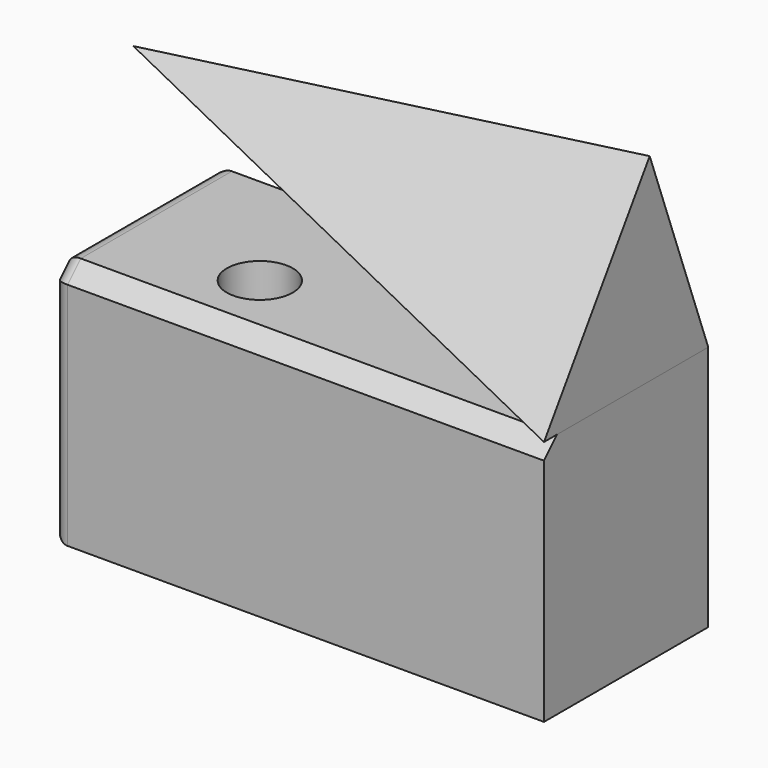
from build123d import *

# Parameters (mm, degrees)
F0_W     = 152.4
F0_H     = 63.5
F1_DEPTH = 76.2
F4_R     = 10.1930298676
F5_DEPTH = 43.23312
F7_SIZE  = 5.08
F8_R     = 5.08


# Not quite as in the source:
# - a feature of the source that left no trace in its solid (it failed there, or was rolled back) is left out


with BuildPart() as f1:
    # F0 (on Top) → F1 (new body)
    with BuildSketch(Plane.XY):
        with Locations((76.2, 31.75)):
            Rectangle(F0_W, F0_H)
    extrude(amount=F1_DEPTH)

    # F4 (on face) → F5 (cut)
    with BuildSketch(Plane.XY.offset(76.2)):
        with Locations((46.0177734494, 23.120848462)):
            Circle(F4_R)
    extrude(amount=-F5_DEPTH, mode=Mode.SUBTRACT)

    # F7
    f7_edges = [f1.edges().sort_by_distance(p)[0] for p in [
        (76.2, 0, 76.2),
    ]]
    chamfer(f7_edges, length=F7_SIZE)

    # F8
    f8_edges = [f1.edges().sort_by_distance(p)[0] for p in [
        (0, 0, 35.56),
        (0, 2.54, 73.66),
        (0, 31.75, 0),
        (0, 34.29, 76.2),
        (0, 63.5, 38.1),
    ]]
    fillet(f8_edges, radius=F8_R)


with BuildPart() as f6:
    # F2 (on face) → F6 section 0
    with BuildSketch(Plane.YZ.offset(152.4), mode=Mode.PRIVATE) as f6_s0:
        Polygon((40.8631898463, 137.4332010746), (0, 76.2), (63.5, 76.2), align=None)
    loft([f6_s0.sketch, Vertex(0, 31.75, 121.5353310108)])


solid = Compound([f1.part, f6.part])
